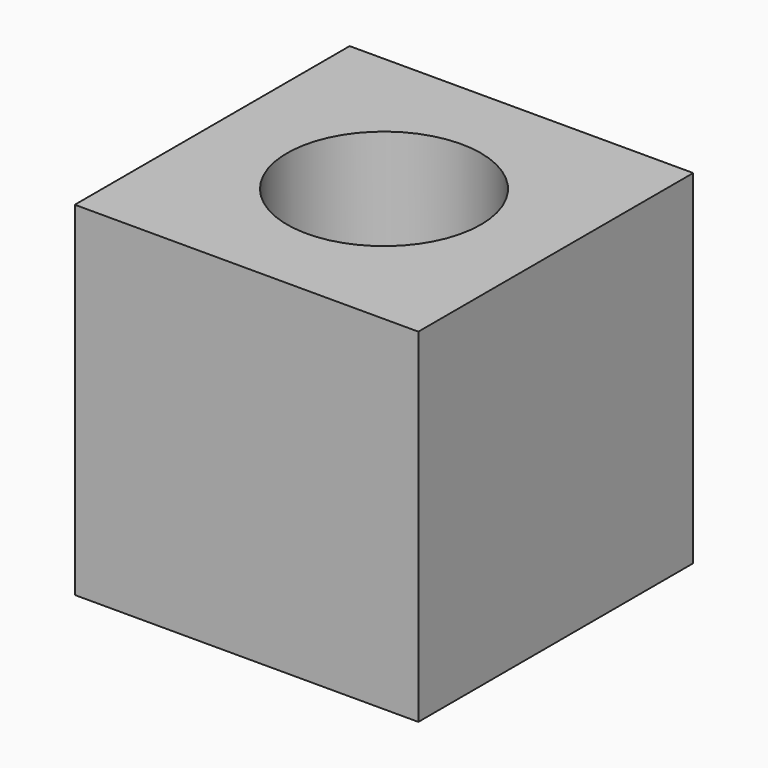
from build123d import *

# Parameters (mm, degrees)
F0_W     = 40
F0_H     = 40
F1_DEPTH = 40
F3_R     = 11.2794780308
F4_DEPTH = 40


# Not quite as in the source:
# - the program builds the solid bodies; features that only make, move or delete a surface that nothing else refers to are left out


with BuildPart() as f1:
    # F0 (on Front) → F1 (new body)
    with BuildSketch(Plane.XZ):
        with Locations((20, 20)):
            Rectangle(F0_W, F0_H)
    extrude(amount=F1_DEPTH)

    # F3 (on face) → F4 (cut)
    with BuildSketch(Plane.XY.offset(40)):
        with Locations((20, -20)):
            Circle(F3_R)
    extrude(amount=-F4_DEPTH, mode=Mode.SUBTRACT)


solid = f1.part
